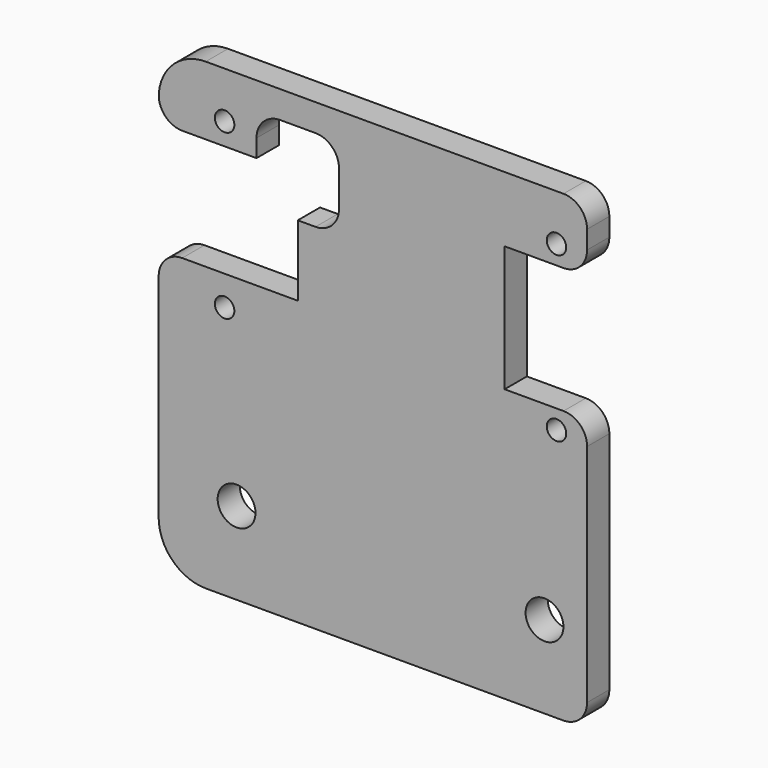
from build123d import *

# Parameters (mm, degrees)
F0_W     = 50
F0_H     = 50
F0_R     = 1.05
F1_DEPTH = 3
F2_W     = 15
F2_H     = 12.085
F3_DEPTH = 3.001
F4_R     = 2.04
F5_DEPTH = 3.001
F7_DEPTH = 3.001
F8_W     = 8.9
F8_H     = 8.9
F9_DEPTH = 3.001
F10_R    = 5.08
F11_R    = 2.54
F12_R    = 2.54


with BuildPart() as f1:
    # F0 (on Front) → F1 (new body)
    with BuildSketch(Plane.XZ):
        with Locations((25, 25)):
            Rectangle(F0_W, F0_H)
        with Locations((7.11, 27.33)):
            Circle(F0_R, mode=Mode.SUBTRACT)
        with Locations((7.11, 45)):
            Circle(F0_R, mode=Mode.SUBTRACT)
        with Locations((42.89, 27.33)):
            Circle(F0_R, mode=Mode.SUBTRACT)
        with Locations((42.89, 45)):
            Circle(F0_R, mode=Mode.SUBTRACT)
    extrude(amount=F1_DEPTH)

    # F2 (on face) → F3 (cut, through all)
    with BuildSketch(Plane.XZ.offset(3)):
        with Locations((7.5, 36.5725)):
            Rectangle(F2_W, F2_H)
    extrude(amount=-F3_DEPTH, mode=Mode.SUBTRACT)

    # F4 (on face) → F5 (cut, through all)
    with BuildSketch(Plane.XZ.offset(3)):
        with Locations((8.4, 8.9)):
            Circle(F4_R)
        with Locations((41.6, 8.9)):
            Circle(F4_R)
    extrude(amount=-F5_DEPTH, mode=Mode.SUBTRACT)

    # F6 (on face) → F7 (cut, through all)
    with BuildSketch(Plane.XZ.offset(3)):
        Polygon((37.3, 29.38), (46.19, 29.38), (46.19, 0), (50, 0), (50, 29.38), (50, 42.95), (50, 50), (46.19, 50), (46.19, 42.95), (37.3, 42.95), align=None)
    extrude(amount=-F7_DEPTH, mode=Mode.SUBTRACT)

    # F8 (on face) → F9 (cut, through all)
    with BuildSketch(Plane(origin=(0, 0, 0), x_dir=(-1, 0, 0), z_dir=(0, 1, 0))):
        with Locations((-15, 42.615)):
            Rectangle(F8_W, F8_H)
    extrude(amount=-F9_DEPTH, mode=Mode.SUBTRACT)

    # F10
    f10_edges = [f1.edges().sort_by_distance(p)[0] for p in [
        (0, -1.5, 50),
        (0, -1.5, 0),
    ]]
    fillet(f10_edges, radius=F10_R)

    # F11
    f11_edges = [f1.edges().sort_by_distance(p)[0] for p in [
        (19.45, -1.5, 47.065),
        (19.45, -1.5, 38.165),
        (10.55, -1.5, 47.065),
    ]]
    fillet(f11_edges, radius=F11_R)

    # F12
    f12_edges = [f1.edges().sort_by_distance(p)[0] for p in [
        (46.19, -1.5, 50),
        (46.19, -1.5, 29.38),
        (46.19, -1.5, 42.95),
        (0, -1.5, 42.615),
        (0, -1.5, 30.53),
        (46.19, -1.5, 0),
    ]]
    fillet(f12_edges, radius=F12_R)


solid = f1.part
